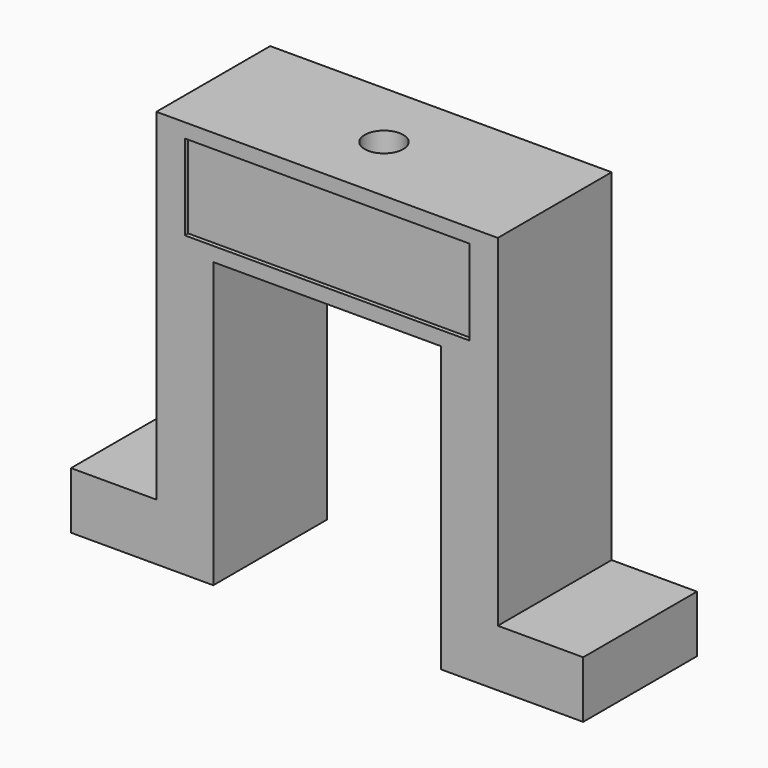
from build123d import *

# Parameters (mm, degrees)
F1_DEPTH = 25
F3_D     = 6.8
F3_DEPTH = 14
F3_TIP   = 2.0429261047
F4_DEPTH = 10
F5_W     = 50
F5_H     = 15
F6_DEPTH = 0.75


with BuildPart() as f1:
    # F0 (on Front) → F1 (new body)
    with BuildSketch(Plane.XZ):
        Polygon((30, 60), (0, 60), (-30, 60), (-30, 10), (-45, 10), (-45, 0), (-20, 0), (-20, 50), (0, 50), (20, 50), (20, 0), (45, 0), (45, 10), (30, 10), align=None)
    extrude(amount=F1_DEPTH)

    # F3
    with Locations(Plane.XY.offset(60)):
        with Locations((0, -12.5)):
            Hole(F3_D / 2, depth=F3_DEPTH)
            with Locations((0, 0, -(F3_DEPTH + F3_TIP / 2))):  # 118° drill point
                Cone(0, F3_D / 2, F3_TIP, mode=Mode.SUBTRACT)

    # F4 (add): a face of the model
    f4_faces = [f1.faces().sort_by_distance(p)[0] for p in [
        (29.35, -12.5, 60),
    ]]
    extrude(f4_faces, amount=F4_DEPTH)

    # F5 (on face) → F6 (cut)
    with BuildSketch(Plane.XZ.offset(25)):
        with Locations((0, 60)):
            Rectangle(F5_W, F5_H)
    extrude(amount=-F6_DEPTH, mode=Mode.SUBTRACT)


solid = f1.part
